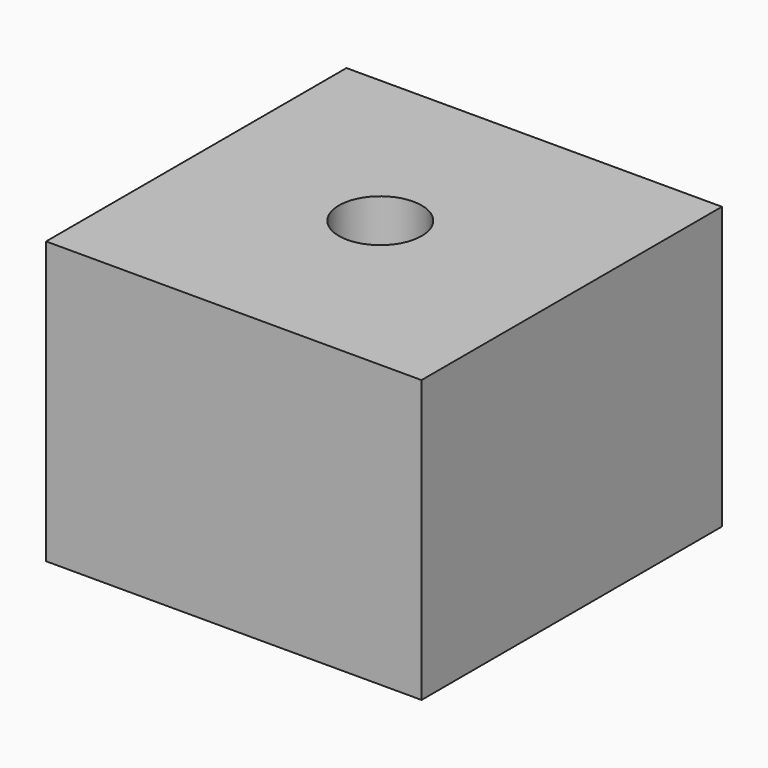
from build123d import *

# Parameters (mm, degrees)
F0_W         = 101.6
F0_H         = 101.6
F1_DEPTH     = 76.2
F3_W         = 101.6
F3_H         = 76.2
F3_TEXT_SIZE = 15.6390144386
F4_DEPTH     = 19.05
F5_TEXT_SIZE = 35.5283729732
F6_DEPTH     = 76.2
F2_R         = 11.1972068222
F7_DEPTH     = 190.5


# Not quite as in the source:
# - Text() gives the source's letters only with a copy of the font that has no kerning and outlines rounded to 1/6400 em; it was checked with that copy


with BuildPart() as f1:
    # F0 (on Top) → F1 (new body)
    with BuildSketch(Plane.XY):
        with Locations((-1.7123259604, 3.535780507)):
            Rectangle(F0_W, F0_H)
    extrude(amount=F1_DEPTH)

    # F3 (on face) → F4 (join)
    with BuildSketch(Plane.YZ.offset(49.0876740396)):
        with Locations((3.535780507, 38.1)):
            Rectangle(F3_W, F3_H)
        Polygon((-2.2528371846, 27.4175982922), (-3.596814988, 27.4175982922), (-4.9872211154, 30.968143289), (-9.4614454024, 30.968143289), (-10.8347463578, 27.4175982922), (-12.1494010091, 27.4175982922), (-7.7362666222, 38.6288167679), (-6.6439792075, 38.6288167679), align=None, mode=Mode.SUBTRACT)
        with Locations((-12.1494010091, 27.4175982922)):
            Text('A', F3_TEXT_SIZE, font='Open Sans', text_align=(TextAlign.LEFT, TextAlign.BOTTOM))
    extrude(amount=-F4_DEPTH)

    # F5 (on face) → F6 (join)
    with BuildSketch(Plane.XZ.offset(47.264219493)):
        with Locations((-4.6839108691, 42.4890890718)):
            Text('E', F5_TEXT_SIZE, font='Open Sans', text_align=(TextAlign.LEFT, TextAlign.BOTTOM))
    extrude(amount=-F6_DEPTH)

    # F2 (on face) → F7 (cut)
    with BuildSketch(Plane.XY.offset(76.2)):
        with Locations((-3.2846704125, 4.2496500537)):
            Circle(F2_R)
    extrude(amount=-F7_DEPTH, mode=Mode.SUBTRACT)


solid = f1.part
